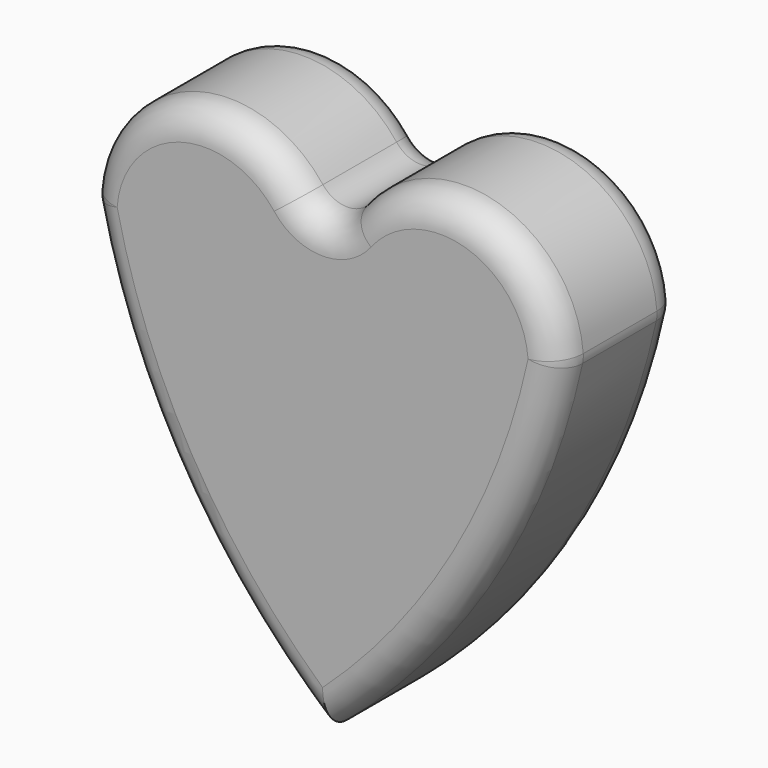
from build123d import *

# Parameters (mm, degrees)
F1_DEPTH = 25.4
F3_R     = 5.08


# Not quite as in the source:
# - a feature of the source that left no trace in its solid (it failed there, or was rolled back) is left out


with BuildPart() as f1:
    # F0 (on Front) → F1 (new body)
    with BuildSketch(Plane.XZ):
        with BuildLine():
            ThreePointArc((39.115998894, 27.4320002645), (20.3391036575, 46.3696241803), (0, 29.1206747426))
            ThreePointArc((0, 29.1206747426), (-20.3391036575, 46.3696241803), (-39.115998894, 27.4320002645))
            ThreePointArc((-39.115998894, 27.4320002645), (-24.9919364346, -8.4631327613), (0, -37.8459990025))
            ThreePointArc((0, -37.8459990025), (24.9919364346, -8.4631327613), (39.115998894, 27.4320002645))
        make_face()
        with BuildLine():
            ThreePointArc((0, 29.1206747426), (0.1433513735, 26.7523380063), (0, 24.3840012699))
            ThreePointArc((0, 24.3840012699), (-0.1433513735, 26.7523380063), (0, 29.1206747426))
        make_face(mode=Mode.SUBTRACT)
        with BuildLine():
            ThreePointArc((0, 29.1206747426), (-0.1433513735, 26.7523380063), (0, 24.3840012699))
            ThreePointArc((0, 24.3840012699), (0.1433513735, 26.7523380063), (0, 29.1206747426))
        make_face()
    extrude(amount=F1_DEPTH)

    # F3
    f3_edges = [f1.edges().sort_by_distance(p)[0] for p in [
        (20.339104, 0, 46.369624),
        (20.339104, -25.4, 46.369624),
        (0, -12.7, 29.120675),
        (-39.115999, -12.7, 27.432),
        (-20.339104, 0, 46.369624),
        (-20.339104, -25.4, 46.369624),
        (39.115999, -12.7, 27.432),
        (-24.991936, 0, -8.463133),
        (-24.991936, -25.4, -8.463133),
        (24.991936, 0, -8.463133),
        (24.991936, -25.4, -8.463133),
    ]]
    fillet(f3_edges, radius=F3_R)


solid = f1.part
